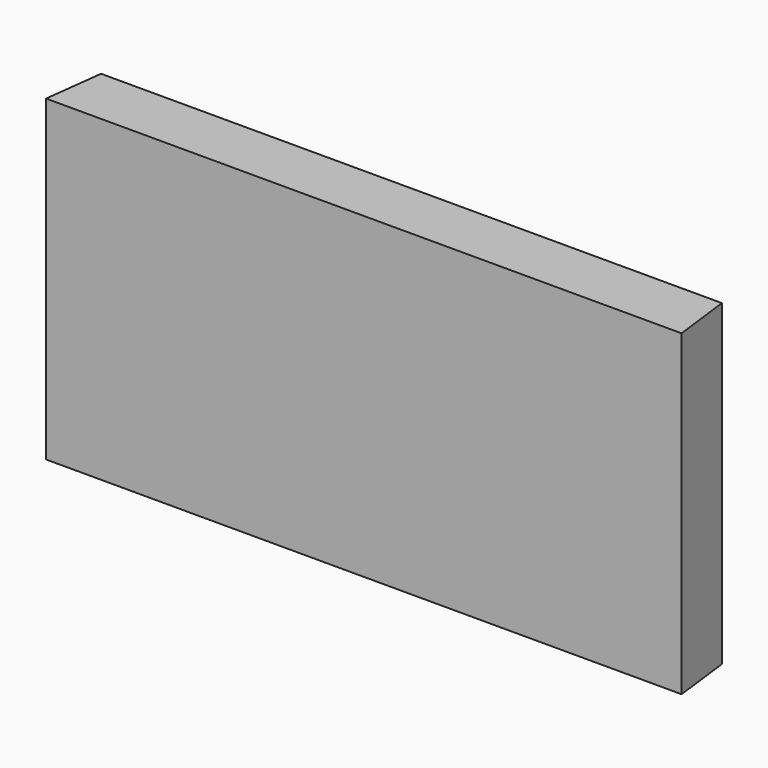
from build123d import *

# Parameters (mm, degrees)
F0_W     = 203.2
F0_H     = 101.6
F1_DEPTH = 19.05
F2_SIZE2 = 2.339036
F2_SIZE  = 19.04999
F3_SIZE2 = 2.339036
F3_SIZE  = 19.04999


# Not quite as in the source:
# - a fillet or chamfer is up to 0.001 mm smaller than in the source, because OpenCascade refuses the exact size


with BuildPart() as f1:
    # F0 (on Front) → F1 (new body)
    with BuildSketch(Plane.XZ):
        Rectangle(F0_W, F0_H)
    extrude(amount=F1_DEPTH)

    # F2 (size 19.05 and 2.3390458852 in the source; OpenCascade refuses exactly that, so slightly less here)
    f2_edges = [f1.edges().sort_by_distance(p)[0] for p in [
        (-101.6, 0, 0),
    ]]
    f2_side = f1.faces().sort_by_distance((-101.6, -9.525, 0))[0]
    chamfer(f2_edges, length=F2_SIZE, length2=F2_SIZE2, reference=f2_side)

    # F3 (size 19.05 and 2.3390458852 in the source; OpenCascade refuses exactly that, so slightly less here)
    f3_edges = [f1.edges().sort_by_distance(p)[0] for p in [
        (101.6, 0, 0),
    ]]
    f3_side = f1.faces().sort_by_distance((101.6, -9.525, 0))[0]
    chamfer(f3_edges, length=F3_SIZE, length2=F3_SIZE2, reference=f3_side)


solid = f1.part
